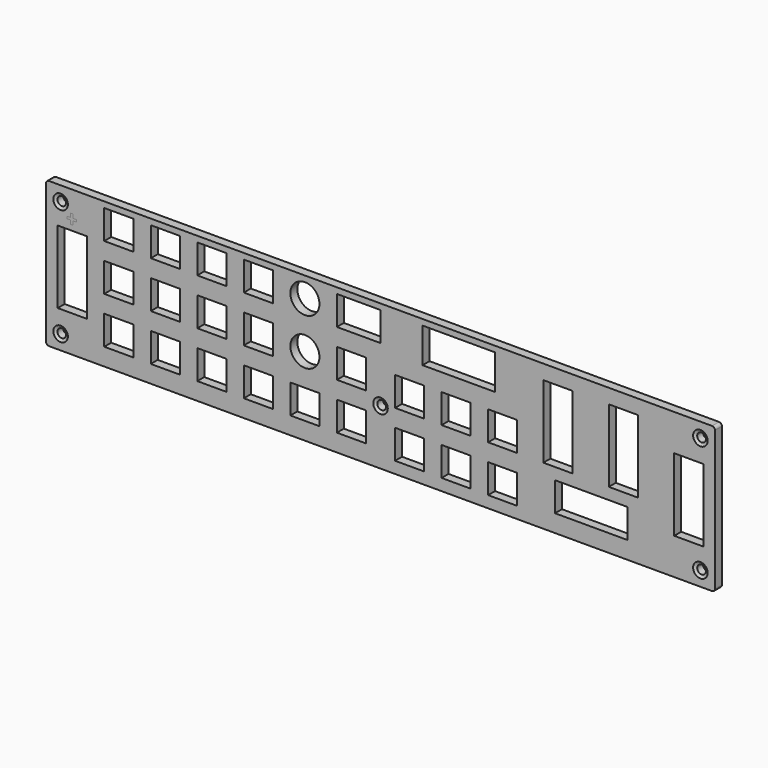
from build123d import *

# Parameters (mm, degrees)
F0_W         = 230
F0_H         = 50
F0_R         = 1.5
F0_W_2       = 10
F0_H_2       = 10
F0_W_3       = 25
F0_H_3       = 25
F0_R_2       = 5
F0_W_4       = 15
F0_H_4       = 12
F1_DEPTH     = 3
F2_SIZE2     = 1
F2_SIZE      = 0.5
F2_2_SIZE2   = 1
F2_2_SIZE    = 0.5
F2_3_SIZE2   = 1
F2_3_SIZE    = 0.5
F2_4_SIZE2   = 1
F2_4_SIZE    = 0.5
F2_5_SIZE2   = 1
F2_5_SIZE    = 0.5
F3_R         = 1
F4_TEXT_SIZE = 7.0183913305
F5_DEPTH     = 1
F6_DEPTH     = 1


# Not quite as in the source:
# - Text() gives the source's letters only with a copy of the font that has no kerning and outlines rounded to 1/6400 em; it was checked with that copy


with BuildPart() as f1:
    # F0 (on Front) → F1 (new body)
    with BuildSketch(Plane.XZ):
        with Locations((0, 9)):
            Rectangle(F0_W, F0_H)
        with Locations((-110, -11)):
            Circle(F0_R, mode=Mode.SUBTRACT)
        with Locations((-90, -5)):
            Rectangle(F0_W_2, F0_H_2, mode=Mode.SUBTRACT)
        with Locations((-74, -5)):
            Rectangle(F0_W_2, F0_H_2, mode=Mode.SUBTRACT)
        with Locations((-58, -5)):
            Rectangle(F0_W_2, F0_H_2, mode=Mode.SUBTRACT)
        with Locations((-42, -5)):
            Rectangle(F0_W_2, F0_H_2, mode=Mode.SUBTRACT)
        with Locations((-26, -5)):
            Rectangle(F0_W_2, F0_H_2, mode=Mode.SUBTRACT)
        with Locations((-10, -5)):
            Rectangle(F0_W_2, F0_H_2, mode=Mode.SUBTRACT)
        with Locations((10, -7)):
            Rectangle(F0_W_2, F0_H_2, mode=Mode.SUBTRACT)
        with Locations((26, -7)):
            Rectangle(F0_W_2, F0_H_2, mode=Mode.SUBTRACT)
        with Locations((42, -7)):
            Rectangle(F0_W_2, F0_H_2, mode=Mode.SUBTRACT)
        with Locations((110, -11)):
            Circle(F0_R, mode=Mode.SUBTRACT)
        with Locations((72.5, -5)):
            Rectangle(F0_W_3, F0_H_2, mode=Mode.SUBTRACT)
        with Locations((0, 3)):
            Circle(F0_R, mode=Mode.SUBTRACT)
        with Locations((-106, 9)):
            Rectangle(F0_W_2, F0_H_3, mode=Mode.SUBTRACT)
        with Locations((-90, 11)):
            Rectangle(F0_W_2, F0_H_2, mode=Mode.SUBTRACT)
        with Locations((-74, 11)):
            Rectangle(F0_W_2, F0_H_2, mode=Mode.SUBTRACT)
        with Locations((-58, 11)):
            Rectangle(F0_W_2, F0_H_2, mode=Mode.SUBTRACT)
        with Locations((-42, 11)):
            Rectangle(F0_W_2, F0_H_2, mode=Mode.SUBTRACT)
        with Locations((-26, 11)):
            Circle(F0_R_2, mode=Mode.SUBTRACT)
        with Locations((-10, 11)):
            Rectangle(F0_W_2, F0_H_2, mode=Mode.SUBTRACT)
        with Locations((-90, 27)):
            Rectangle(F0_W_2, F0_H_2, mode=Mode.SUBTRACT)
        with Locations((-74, 27)):
            Rectangle(F0_W_2, F0_H_2, mode=Mode.SUBTRACT)
        with Locations((-58, 27)):
            Rectangle(F0_W_2, F0_H_2, mode=Mode.SUBTRACT)
        with Locations((-110, 29)):
            Circle(F0_R, mode=Mode.SUBTRACT)
        with Locations((-42, 27)):
            Rectangle(F0_W_2, F0_H_2, mode=Mode.SUBTRACT)
        with Locations((-26, 27)):
            Circle(F0_R_2, mode=Mode.SUBTRACT)
        with Locations((-7.5, 27)):
            Rectangle(F0_W_4, F0_H_2, mode=Mode.SUBTRACT)
        with Locations((10, 9)):
            Rectangle(F0_W_2, F0_H_2, mode=Mode.SUBTRACT)
        with Locations((26, 9)):
            Rectangle(F0_W_2, F0_H_2, mode=Mode.SUBTRACT)
        with Locations((42, 9)):
            Rectangle(F0_W_2, F0_H_2, mode=Mode.SUBTRACT)
        with Locations((106, 9)):
            Rectangle(F0_W_2, F0_H_3, mode=Mode.SUBTRACT)
        with Locations((61, 16.5)):
            Rectangle(F0_W_2, F0_H_3, mode=Mode.SUBTRACT)
        with Locations((83.5, 16.5)):
            Rectangle(F0_W_2, F0_H_3, mode=Mode.SUBTRACT)
        with Locations((26.9479073584, 26)):
            Rectangle(F0_W_3, F0_H_4, mode=Mode.SUBTRACT)
        with Locations((110, 29)):
            Circle(F0_R, mode=Mode.SUBTRACT)
    extrude(amount=F1_DEPTH)

    # F2
    f2_edges = [f1.edges().sort_by_distance(p)[0] for p in [
        (-111.5, -3, 29),
    ]]
    f2_side = f1.faces().sort_by_distance((-111.5, -1.5, 29))[0]
    chamfer(f2_edges, length=F2_SIZE, length2=F2_SIZE2, reference=f2_side)

    # F2#2
    f2_2_edges = [f1.edges().sort_by_distance(p)[0] for p in [
        (-111.5, -3, -11),
    ]]
    f2_2_side = f1.faces().sort_by_distance((-111.5, -1.5, -11))[0]
    chamfer(f2_2_edges, length=F2_2_SIZE, length2=F2_2_SIZE2, reference=f2_2_side)

    # F2#3
    f2_3_edges = [f1.edges().sort_by_distance(p)[0] for p in [
        (-1.5, -3, 3),
    ]]
    f2_3_side = f1.faces().sort_by_distance((-1.5, -1.5, 3))[0]
    chamfer(f2_3_edges, length=F2_3_SIZE, length2=F2_3_SIZE2, reference=f2_3_side)

    # F2#4
    f2_4_edges = [f1.edges().sort_by_distance(p)[0] for p in [
        (108.5, -3, -11),
    ]]
    f2_4_side = f1.faces().sort_by_distance((108.5, -1.5, -11))[0]
    chamfer(f2_4_edges, length=F2_4_SIZE, length2=F2_4_SIZE2, reference=f2_4_side)

    # F2#5
    f2_5_edges = [f1.edges().sort_by_distance(p)[0] for p in [
        (108.5, -3, 29),
    ]]
    f2_5_side = f1.faces().sort_by_distance((108.5, -1.5, 29))[0]
    chamfer(f2_5_edges, length=F2_5_SIZE, length2=F2_5_SIZE2, reference=f2_5_side)

    # F3
    f3_edges = [f1.edges().sort_by_distance(p)[0] for p in [
        (-115, -1.5, 34),
        (-115, -1.5, -16),
        (115, -1.5, -16),
        (115, -1.5, 34),
    ]]
    fillet(f3_edges, radius=F3_R)

    # F4 (on face) → F5 (cut)
    with BuildSketch(Plane.XZ.offset(3)):
        with Locations((-108.159493487, 22.5)):
            Text('+', F4_TEXT_SIZE, font='Open Sans', font_style=FontStyle.BOLD, text_align=(TextAlign.LEFT, TextAlign.BOTTOM))
    extrude(amount=-F5_DEPTH, mode=Mode.SUBTRACT)


with BuildPart() as f6:
    # F6 (new): a face of the model
    f6_faces = [f1.part.faces().sort_by_distance(p)[0] for p in [
        (-106.1565103987, -2, 24.9775144488),
    ]]
    extrude(f6_faces, amount=F6_DEPTH)


solid = Compound([f1.part, f6.part])
